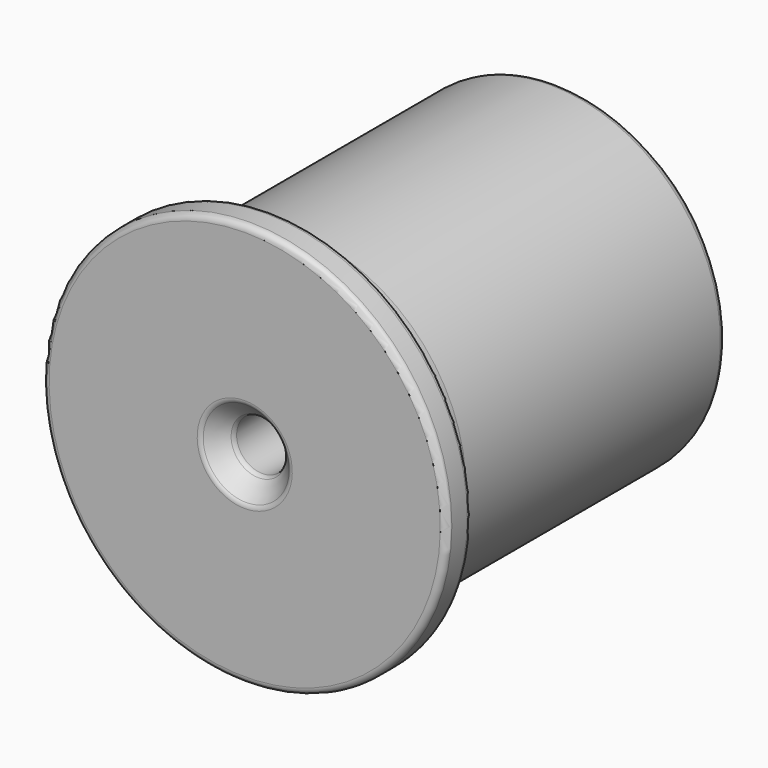
from build123d import *

# Parameters (mm, degrees)
F0_W    = 58
F0_H    = 22.5
F2_SIZE = 3
F4_R    = 1


# Not quite as in the source:
# - a fillet or chamfer that OpenCascade refuses, or shapes differently, is made with other operations: its cross-section is extruded or revolved along the edge and cut away or added


with BuildPart() as f1:
    # F0 (on Right) → F1 (revolve)
    with BuildSketch(Plane.YZ):
        Polygon((0, 31.5), (0, 4), (5, 4), (5, 26.5), (5, 31.5), align=None)
        with Locations((34, 15.25)):
            Rectangle(F0_W, F0_H)
    revolve(axis=Axis((0, 38.0806664313, 0), (0, 1, 0)))

    # F2
    f2_edges = [f1.edges().sort_by_distance(p)[0] for p in [
        (0, 63, -26.5),
        (0, 63, -4),
        (0, 0, -4),
    ]]
    chamfer(f2_edges, length=F2_SIZE)

    # F3: chamfer of 5 x 0.5 on 1 edges, made by hand

    # F3_s1 → F3_t2 (revolve)
    with BuildSketch(Plane.YZ):
        Polygon((5, 27), (10, 26.5), (5, 26.5), align=None)
    revolve(axis=Axis((0, 5, 0), (0, 1, 0)))

    # F4
    f4_edges = [f1.edges().sort_by_distance(p)[0] for p in [
        (0, 0, -31.5),
        (0, 5, -31.5),
        (0, 5, -27),
        (0, 60, -26.5),
        (0, 63, -23.5),
        (0, 60, -4),
        (0, 63, -7),
        (0, 0, -7),
        (0, 3, -4),
    ]]
    fillet(f4_edges, radius=F4_R)


solid = f1.part
